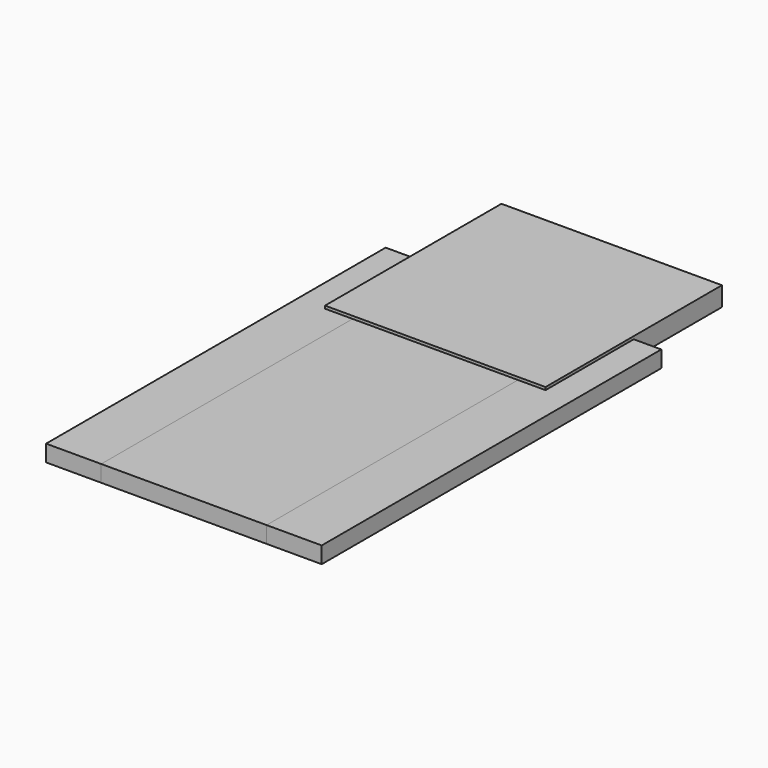
from build123d import *

# Parameters (mm, degrees)
F0_W     = 500
F0_H     = 30
F1_DEPTH = 770
F2_W     = 400
F2_H     = 400
F3_DEPTH = 20
F4_W     = 400
F4_H     = 400
F4_W_2   = 180
F4_H_2   = 180
F5_DEPTH = 15
F6_W     = 300
F6_H     = 30
F7_DEPTH = 770


with BuildPart() as f1:
    # F0 (on Front) → F1 (new body)
    with BuildSketch(Plane.XZ):
        Rectangle(F0_W, F0_H)
    extrude(amount=F1_DEPTH)


with BuildPart() as f3:
    # F2 (on Top) → F3 (new body)
    with BuildSketch(Plane.XY):
        Rectangle(F2_W, F2_H)
    extrude(amount=F3_DEPTH)

    # F4 (on face) → F5 (join)
    with BuildSketch(Plane(origin=(0, 0, 0), x_dir=(1, 0, 0), z_dir=(0, 0, -1))):
        Rectangle(F4_W, F4_H)
        Rectangle(F4_W_2, F4_H_2, mode=Mode.SUBTRACT)
    extrude(amount=F5_DEPTH)


with BuildPart() as f7:
    # F6 (on Front) → F7 (new body)
    with BuildSketch(Plane.XZ):
        Rectangle(F6_W, F6_H)
    extrude(amount=F7_DEPTH)


solid = Compound([f1.part, f3.part, f7.part])
